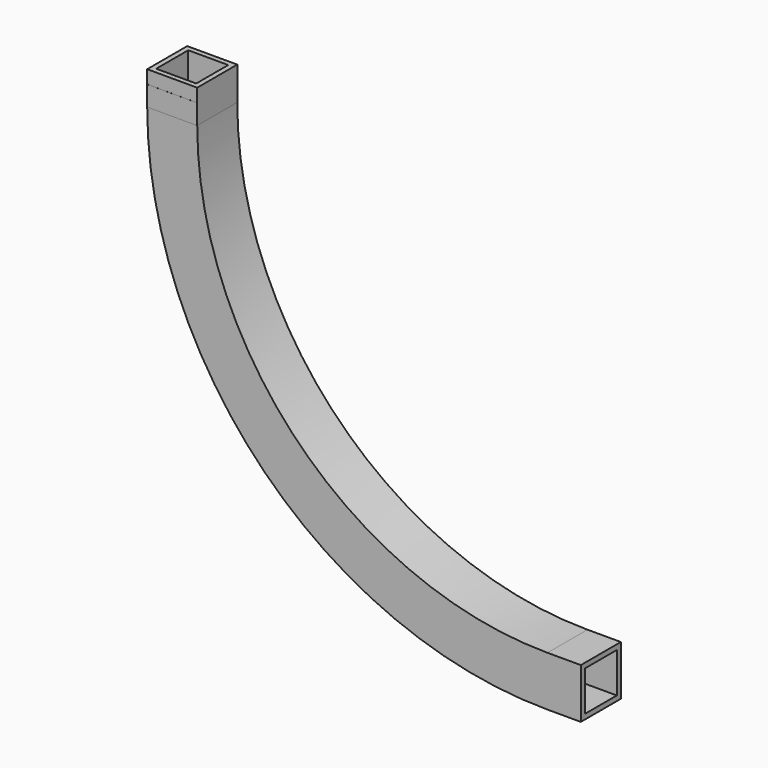
from build123d import *

# Parameters (mm, degrees)
F1_DEPTH = 15
F2_DEPTH = 10
F3_DEPTH = 10
F4_W     = 15
F4_H     = 10
F5_DEPTH = 0.01
F6_W     = 15
F6_H     = 4
F7_DEPTH = 0.01
F8_W     = 12
F8_H     = 12


with BuildPart() as f1:
    # F0 (on Front) → F1 (new body)
    with BuildSketch(Plane.XZ):
        with BuildLine():
            Line((-105, 0), (-120, 0))
            ThreePointArc((-120, 0), (-84.8528137424, -84.8528137424), (0, -120))
            Line((0, -120), (0, -105))
            ThreePointArc((0, -105), (-74.2462120246, -74.2462120246), (-105, 0))
        make_face()
    extrude(amount=F1_DEPTH)

    # F2 (add): a face of the model
    f2_faces = [f1.faces().sort_by_distance(p)[0] for p in [
        (-112.5, -7.5, 0),
    ]]
    extrude(f2_faces, amount=F2_DEPTH)

    # F3 (add): a face of the model
    f3_faces = [f1.faces().sort_by_distance(p)[0] for p in [
        (0, -7.5, -112.5),
    ]]
    extrude(f3_faces, amount=F3_DEPTH)

    # F4 (on face) → F5 (join)
    with BuildSketch(Plane.XZ.offset(15)):
        with Locations((-112.5, 5)):
            Rectangle(F4_W, F4_H)
    extrude(amount=F5_DEPTH)

    # F6 (on face) → F7 (cut)
    with BuildSketch(Plane.XZ.offset(15.01)):
        with Locations((-112.5, 8)):
            Rectangle(F6_W, F6_H)
    extrude(amount=-F7_DEPTH, mode=Mode.SUBTRACT)

    # F9: sweep along a path in F9_path
    with BuildLine(Plane(origin=(-105, 0, 0), x_dir=(0, 0, -1), z_dir=(0, 1, 0))) as f9_path:
        Line((-10, 0), (0, 0))
        ThreePointArc((0, 0), (74.2462120246, -30.7537879754), (105, -105))
        Line((105, -105), (105, -115))
    # F8 (on face) → F9 (sweep, cut)
    with BuildSketch(Plane.YZ.offset(10)):
        with Locations((-7.5, -112.5)):
            Rectangle(F8_W, F8_H)
    sweep(path=f9_path.line, mode=Mode.SUBTRACT)


solid = f1.part
